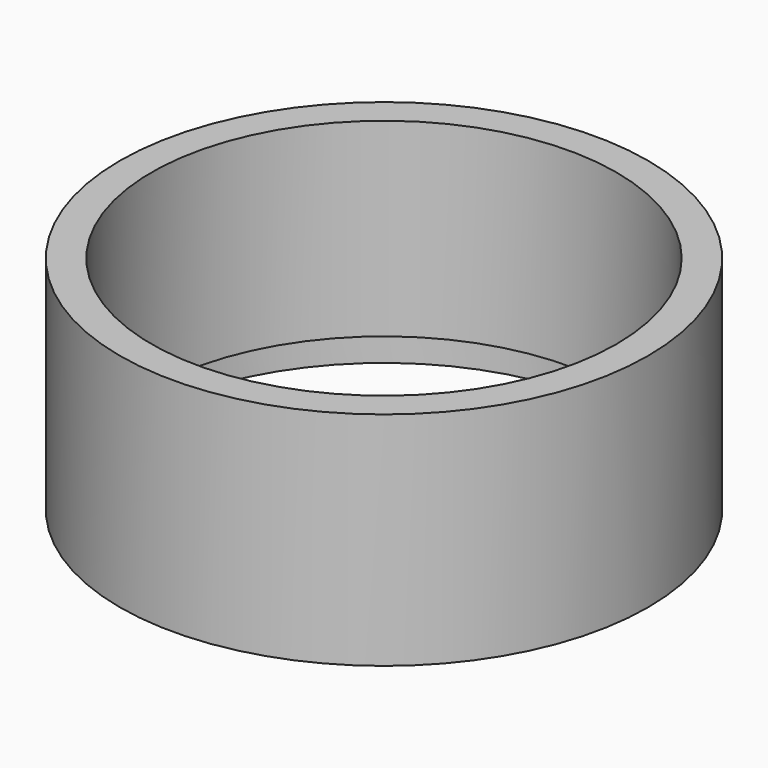
from build123d import *

# Parameters (mm, degrees)
F0_R     = 83.5
F0_R_2   = 78.5
F0_R_3   = 73.5
F1_DEPTH = 60
F2_DEPTH = 10


# Not quite as in the source:
# - a feature of the source that left no trace in its solid (it failed there, or was rolled back) is left out


with BuildPart() as f1:
    # F0 (on Top) → F1 (new body)
    with BuildSketch(Plane.XY):
        Circle(F0_R)
        Circle(F0_R_2, mode=Mode.SUBTRACT)
        Circle(F0_R_2)
        Circle(F0_R_3, mode=Mode.SUBTRACT)
    extrude(amount=F1_DEPTH)

    # F0 (on Top) → F2 (join)
    with BuildSketch(Plane.XY):
        Circle(F0_R)
        Circle(F0_R_2, mode=Mode.SUBTRACT)
    extrude(amount=-F2_DEPTH)


solid = f1.part
